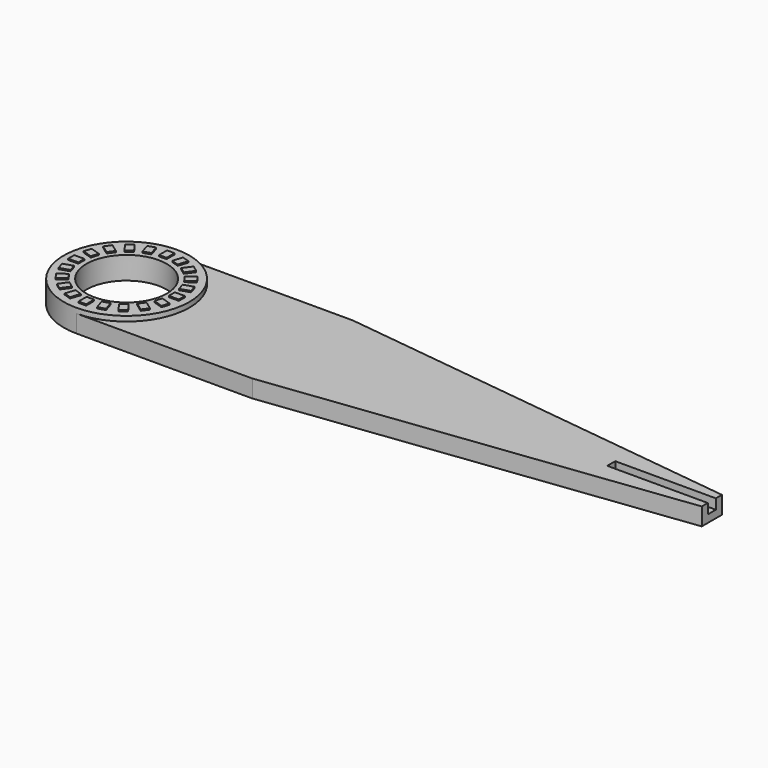
from build123d import *

# Parameters (mm, degrees)
F0_R         = 8
F1_DEPTH     = 3.5
F2_R         = 12.5
F2_R_2       = 8
F3_DEPTH     = 1
F4_W         = 1.5
F4_H         = 2
F4_W_2       = 2
F4_H_2       = 1.5
F5_DEPTH     = 0.25
F6_W         = 20
F6_H         = 2
F7_DEPTH     = 2
F8_TEXT_SIZE = 11.207306266
F9_DEPTH     = 1


# Not quite as in the source:
# - Text() gives the source's letters only with a copy of the font that has no kerning and outlines rounded to 1/6400 em; it was checked with that copy


with BuildPart() as f1:
    # F0 (on Top) → F1 (new body)
    with BuildSketch(Plane.XY):
        with BuildLine():
            Line((35, 12.5), (0, 12.5))
            ThreePointArc((0, 12.5), (-12.5, 0), (0, -12.5))
            Line((0, -12.5), (35, -12.5))
            Line((35, -12.5), (116.3887844346, -2.5067138408))
            Line((116.3887844346, -2.5067138408), (116.3887844346, 2.5067138408))
            Line((116.3887844346, 2.5067138408), (35, 12.5))
        make_face()
        Circle(F0_R, mode=Mode.SUBTRACT)
    extrude(amount=F1_DEPTH)

    # F2 (on face) → F3 (join)
    with BuildSketch(Plane.XY.offset(3.5)):
        Circle(F2_R)
        Circle(F2_R_2, mode=Mode.SUBTRACT)
    extrude(amount=F3_DEPTH)

    # F4 (on face) → F5 (join)
    with BuildSketch(Plane.XY.offset(4.5)):
        with Locations((0, 10)):
            Rectangle(F4_W, F4_H)
        Polygon((-2.6858945509, 10.693384425), (-4.1124793253, 10.2298589335), (-3.4944453366, 8.3277459009), (-2.0678605622, 8.7912713924), align=None)
        Polygon((-5.8588750294, 9.3400258773), (-7.072400521, 8.4583479989), (-5.8968300164, 6.8403140102), (-4.6833045249, 7.7219918886), align=None)
        Polygon((-8.4583479989, 7.072400521), (-9.3400258773, 5.8588750294), (-7.7219918886, 4.6833045249), (-6.8403140102, 5.8968300164), align=None)
        Polygon((-10.2298589335, 4.1124793253), (-10.693384425, 2.6858945509), (-8.7912713924, 2.0678605622), (-8.3277459009, 3.4944453366), align=None)
        with Locations((-10, 0)):
            Rectangle(F4_W_2, F4_H_2)
        Polygon((-10.693384425, -2.6858945509), (-10.2298589335, -4.1124793253), (-8.3277459009, -3.4944453366), (-8.7912713924, -2.0678605622), align=None)
        Polygon((-9.3400258773, -5.8588750294), (-8.4583479989, -7.072400521), (-6.8403140102, -5.8968300164), (-7.7219918886, -4.6833045249), align=None)
        Polygon((-7.072400521, -8.4583479989), (-5.8588750294, -9.3400258773), (-4.6833045249, -7.7219918886), (-5.8968300164, -6.8403140102), align=None)
        Polygon((-4.1124793253, -10.2298589335), (-2.6858945509, -10.693384425), (-2.0678605622, -8.7912713924), (-3.4944453366, -8.3277459009), align=None)
        with Locations((0, -10)):
            Rectangle(F4_W, F4_H)
        Polygon((2.6858945509, -10.693384425), (4.1124793253, -10.2298589335), (3.4944453366, -8.3277459009), (2.0678605622, -8.7912713924), align=None)
        Polygon((5.8588750294, -9.3400258773), (7.072400521, -8.4583479989), (5.8968300164, -6.8403140102), (4.6833045249, -7.7219918886), align=None)
        Polygon((8.4583479989, -7.072400521), (9.3400258773, -5.8588750294), (7.7219918886, -4.6833045249), (6.8403140102, -5.8968300164), align=None)
        Polygon((10.2298589335, -4.1124793253), (10.693384425, -2.6858945509), (8.7912713924, -2.0678605622), (8.3277459009, -3.4944453366), align=None)
        with Locations((10, 0)):
            Rectangle(F4_W_2, F4_H_2)
        Polygon((10.693384425, 2.6858945509), (10.2298589335, 4.1124793253), (8.3277459009, 3.4944453366), (8.7912713924, 2.0678605622), align=None)
        Polygon((9.3400258773, 5.8588750294), (8.4583479989, 7.072400521), (6.8403140102, 5.8968300164), (7.7219918886, 4.6833045249), align=None)
        Polygon((7.072400521, 8.4583479989), (5.8588750294, 9.3400258773), (4.6833045249, 7.7219918886), (5.8968300164, 6.8403140102), align=None)
        Polygon((4.1124793253, 10.2298589335), (2.6858945509, 10.693384425), (2.0678605622, 8.7912713924), (3.4944453366, 8.3277459009), align=None)
    extrude(amount=F5_DEPTH)

    # F6 (on face) → F7 (cut)
    with BuildSketch(Plane.XY.offset(3.5)):
        with Locations((106.3887844346, -0.0067138408)):
            Rectangle(F6_W, F6_H)
    extrude(amount=-F7_DEPTH, mode=Mode.SUBTRACT)

    # F8 (on face) → F9 (join)
    with BuildSketch(Plane(origin=(0, 0, 0), x_dir=(1, 0, 0), z_dir=(0, 0, -1))):
        with Locations((20.3955313191, -4.0346300229)):
            Text('Leann', F8_TEXT_SIZE, font='Open Sans', text_align=(TextAlign.LEFT, TextAlign.BOTTOM))
    extrude(amount=F9_DEPTH)


solid = f1.part
